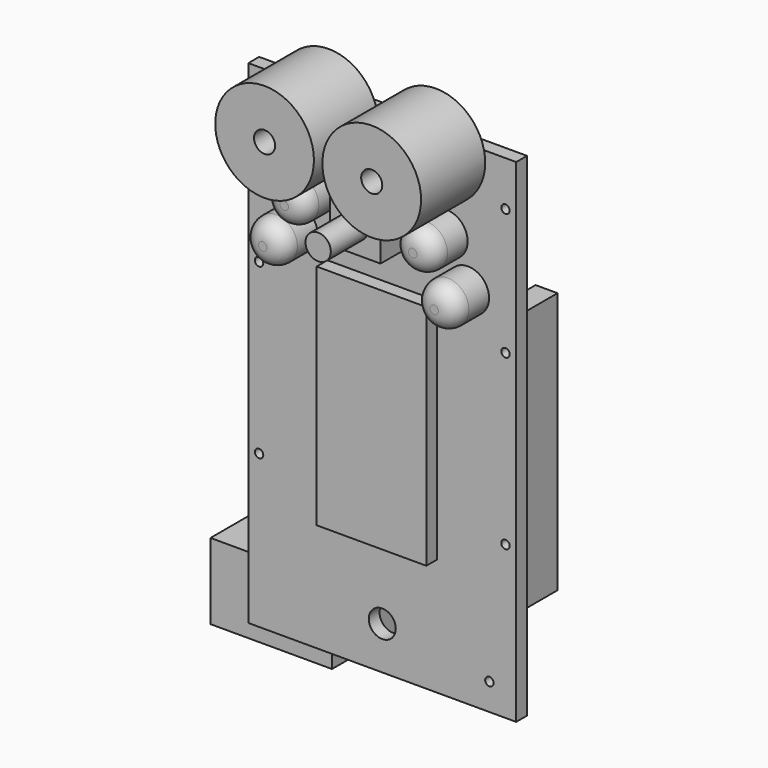
from build123d import *

# Parameters (mm, degrees)
F0_W      = 31.75
F0_H      = 58.42
F0_R      = 0.5
F0_R_2    = 1.6
F1_DEPTH  = 1.6
F2_W      = 6
F2_H      = 6
F3_DEPTH  = 4
F4_R      = 1.5
F5_DEPTH  = 9.5
F6_R      = 5.85
F7_DEPTH  = 9.5
F8_W      = 13
F8_H      = 27
F9_DEPTH  = 1.6
F10_W     = 18.7
F10_H     = 34
F11_DEPTH = 4
F12_W     = 2.6
F12_H     = 31
F13_DEPTH = 8.45
F14_W     = 14.4
F14_H     = 9
F15_DEPTH = 11
F16_W     = 12.3
F16_H     = 2
F17_DEPTH = 5
F18_R     = 2.5
F19_DEPTH = 5
F20_R     = 2
F21_R     = 1.25
F22_DEPTH = 3


with BuildPart() as f1:
    # F0 (on Front) → F1 (new body)
    with BuildSketch(Plane.XZ):
        with Locations((0, -19.05)):
            Rectangle(F0_W, F0_H)
        with Locations((-14.605, -30.16)):
            Circle(F0_R, mode=Mode.SUBTRACT)
        with Locations((0, -43.18)):
            Circle(F0_R_2, mode=Mode.SUBTRACT)
        with Locations((12.7, -45.085)):
            Circle(F0_R, mode=Mode.SUBTRACT)
        with Locations((14.605, -30.16)):
            Circle(F0_R, mode=Mode.SUBTRACT)
        with Locations((-14.605, -10.16)):
            Circle(F0_R, mode=Mode.SUBTRACT)
        with Locations((-14.605, 4.84)):
            Circle(F0_R, mode=Mode.SUBTRACT)
        with Locations((14.605, -10.16)):
            Circle(F0_R, mode=Mode.SUBTRACT)
        with Locations((14.605, 4.84)):
            Circle(F0_R, mode=Mode.SUBTRACT)
    extrude(amount=-F1_DEPTH)

    # F2 (on Front) → F3 (join)
    with BuildSketch(Plane.XZ):
        Rectangle(F2_W, F2_H)
    extrude(amount=F3_DEPTH)

    # F4 (on Front) → F5 (join)
    with BuildSketch(Plane.XZ):
        Circle(F4_R)
    extrude(amount=F5_DEPTH)

    # F6 (on Front) → F7 (join)
    with BuildSketch(Plane.XZ):
        with Locations((-6.35, 8.89)):
            Circle(F6_R)
        with Locations((6.35, 8.89)):
            Circle(F6_R)
    extrude(amount=F7_DEPTH)

    # F8 (on Front) → F9 (join)
    with BuildSketch(Plane.XZ):
        with Locations((0, -20.866)):
            Rectangle(F8_W, F8_H)
    extrude(amount=F9_DEPTH)

    # F18 (on Front) → F19 (join)
    with BuildSketch(Plane.XZ):
        with Locations((-7.62, 0)):
            Circle(F18_R)
        with Locations((7.62, 0)):
            Circle(F18_R)
        with Locations((10.16, -5.08)):
            Circle(F18_R)
        with Locations((-10.16, -5.08)):
            Circle(F18_R)
    extrude(amount=F19_DEPTH)

    # F20
    f20_edges = [f1.edges().sort_by_distance(p)[0] for p in [
        (-12.66, -5, -5.08),
        (-10.12, -5, 0),
        (5.12, -5, 0),
        (7.66, -5, -5.08),
    ]]
    fillet(f20_edges, radius=F20_R)

    # F21 (on face) → F22 (cut)
    with BuildSketch(Plane.XZ.offset(9.5)):
        with Locations((-6.35, 8.89)):
            Circle(F21_R)
        with Locations((6.35, 8.89)):
            Circle(F21_R)
    extrude(amount=-F22_DEPTH, mode=Mode.SUBTRACT)


with BuildPart() as f11:
    # F10 (on face) → F11 (new body)
    with BuildSketch(Plane(origin=(0, 1.6, 0), x_dir=(-1, 0, 0), z_dir=(0, 1, 0))):
        with Locations((0, -23.35)):
            Rectangle(F10_W, F10_H)
    extrude(amount=F11_DEPTH)


with BuildPart() as f13:
    # F12 (on face) → F13 (new body)
    with BuildSketch(Plane(origin=(0, 1.6, 0), x_dir=(-1, 0, 0), z_dir=(0, 1, 0))):
        with Locations((-11.43, -24.13)):
            Rectangle(F12_W, F12_H)
    extrude(amount=F13_DEPTH)


with BuildPart() as f13b:
    # F12 (on face) → F13, piece 2 (new body)
    with BuildSketch(Plane(origin=(0, 1.6, 0), x_dir=(-1, 0, 0), z_dir=(0, 1, 0))):
        with Locations((11.43, -24.13)):
            Rectangle(F12_W, F12_H)
    extrude(amount=F13_DEPTH)


with BuildPart() as f15:
    # F14 (on face) → F15 (new body)
    with BuildSketch(Plane(origin=(0, 1.6, 0), x_dir=(-1, 0, 0), z_dir=(0, 1, 0))):
        with Locations((14.439, -46.41)):
            Rectangle(F14_W, F14_H)
    extrude(amount=F15_DEPTH)


with BuildPart() as f17:
    # F16 (on face) → F17 (new body)
    with BuildSketch(Plane(origin=(0, 1.6, 0), x_dir=(-1, 0, 0), z_dir=(0, 1, 0))):
        with Locations((0, -5.08)):
            Rectangle(F16_W, F16_H)
    extrude(amount=F17_DEPTH)


solid = Compound([f1.part, f11.part, f13.part, f13b.part, f15.part, f17.part])
